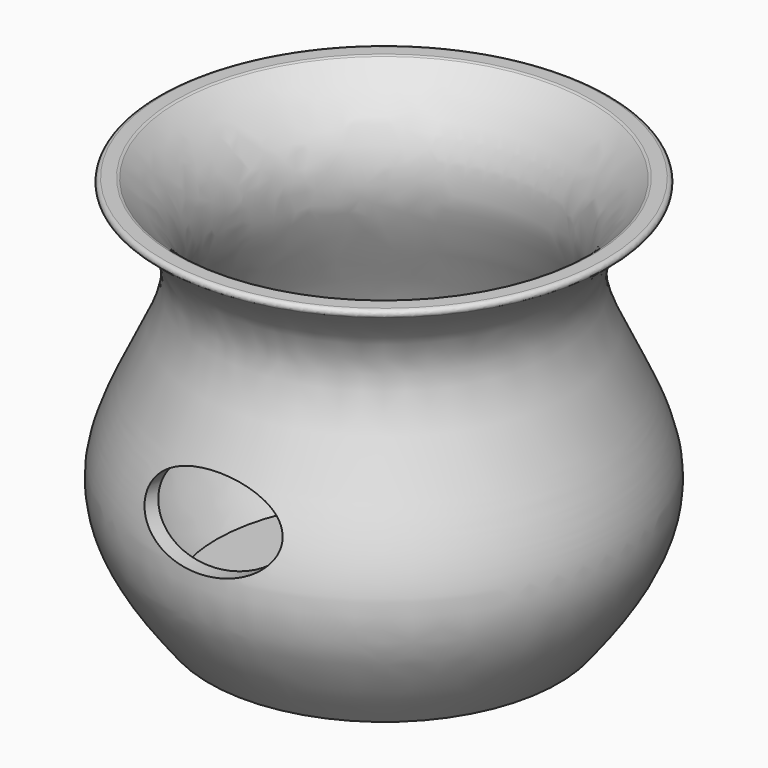
from build123d import *

# Parameters (mm, degrees)
F2_T     = -4
F3_R     = 1
F6_DEPTH = 30


with BuildPart() as f1:
    # F0 (on Front) → F1 (revolve)
    with BuildSketch(Plane.XZ):
        with BuildLine():
            Line((-45, 0), (0, 0))
            Line((0, 0), (0, 100))
            Line((0, 100), (-60, 100))
            add(Edge.make_bspline(
                [(-60, 100), (-48.6602336168, 91.8186455965), (-37.2091677611, 75.8083467752), (-69.5047725932, 34.2279575992), (-53.7829734385, 11.1355138943), (-45, 0)],
                knots=[0, 0, 0, 0, 0.2982106568, 0.6591914917, 1, 1, 1, 1], degree=3))
        make_face()
    revolve(axis=Axis((0, 0, 50), (0, 0, 1)))

    # F2
    f2_openings = [f1.faces().sort_by_distance(p)[0] for p in [
        (0, 0, 100),
    ]]
    offset(amount=F2_T, openings=f2_openings)

    # F3
    f3_edges = [f1.edges().sort_by_distance(p)[0] for p in [
        (60, 0, 100),
        (53.424445, 0, 100),
    ]]
    fillet(f3_edges, radius=F3_R)

    # F5 (on offset) → F6 (cut)
    with BuildSketch(Plane.XZ.offset(70)):
        with BuildLine():
            add(Edge.make_bspline(
                [(17.5, 44.7022020817), (17.5, 62.0227101574), (-8.75, 53.3624561195), (-35, 44.7022020817), (-8.75, 36.0419480438), (17.5, 27.381694006), (17.5, 44.7022020817)],
                knots=[0, 0, 0, 2.0943951024, 2.0943951024, 4.1887902048, 4.1887902048, 6.2831853072, 6.2831853072, 6.2831853072], degree=2, weights=[1, 0.5, 1, 0.5, 1, 0.5, 1]))
        make_face()
    extrude(amount=-F6_DEPTH, mode=Mode.SUBTRACT)


solid = f1.part
